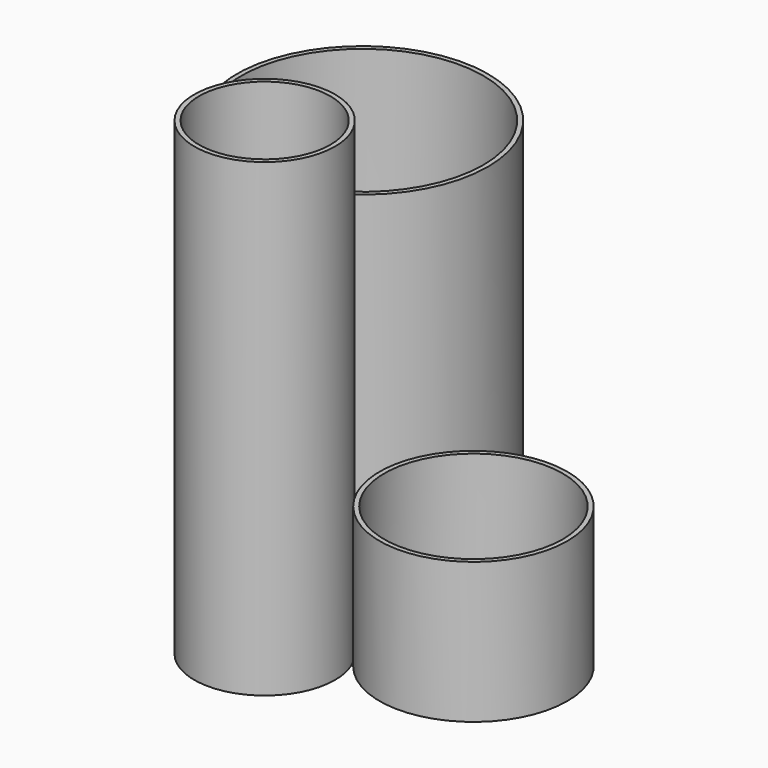
from build123d import *

# Parameters (mm, degrees)
F0_R     = 20
F1_DEPTH = 30
F2_T     = -1
F3_R     = 26.75
F4_DEPTH = 80
F5_T     = -1
F6_R     = 15
F7_DEPTH = 100
F8_T     = -1


with BuildPart() as f1:
    # F0 (on Top) → F1 (new body)
    with BuildSketch(Plane.XY):
        Circle(F0_R)
    extrude(amount=F1_DEPTH)

    # F2
    f2_openings = [f1.faces().sort_by_distance(p)[0] for p in [
        (0, 0, 30),
    ]]
    offset(amount=F2_T, openings=f2_openings)


with BuildPart() as f4:
    # F3 (on Top) → F4 (new body)
    with BuildSketch(Plane.XY):
        with Locations((-41.25, 22)):
            Circle(F3_R)
    extrude(amount=F4_DEPTH)

    # F5
    f5_openings = [f4.faces().sort_by_distance(p)[0] for p in [
        (-41.25, 22, 80),
    ]]
    offset(amount=F5_T, openings=f5_openings)


with BuildPart() as f7:
    # F6 (on Top) → F7 (new body)
    with BuildSketch(Plane.XY):
        with Locations((-29.9080578136, -18.1798811277)):
            Circle(F6_R)
    extrude(amount=F7_DEPTH)

    # F8
    f8_openings = [f7.faces().sort_by_distance(p)[0] for p in [
        (-29.908058, -18.179881, 100),
    ]]
    offset(amount=F8_T, openings=f8_openings)


solid = Compound([f1.part, f4.part, f7.part])
